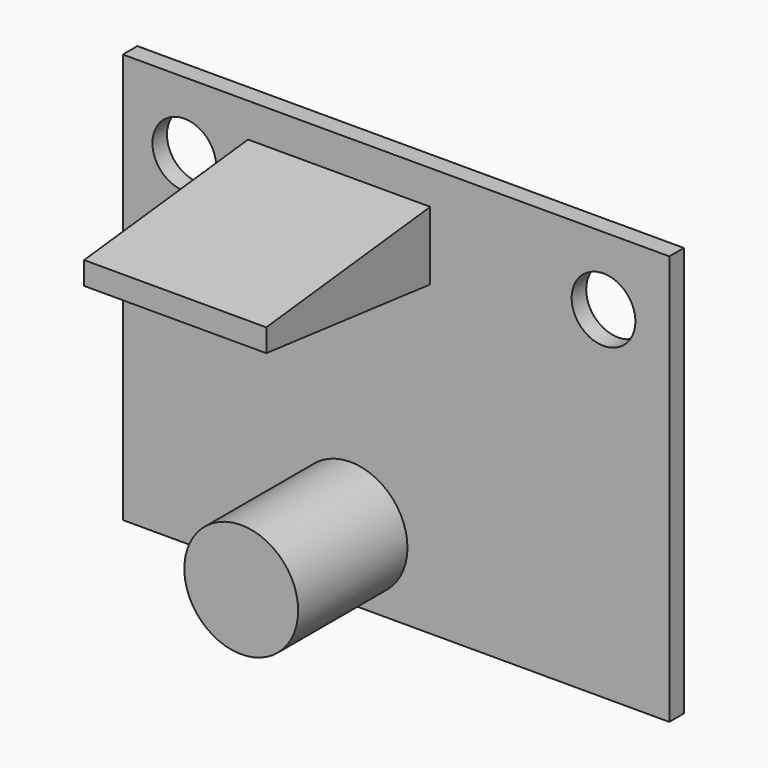
from build123d import *

# Parameters (mm, degrees)
F0_W     = 24
F0_H     = 18
F0_R     = 2.5
F0_W_2   = 8
F0_H_2   = 3
F1_DEPTH = 0.8
F2_D     = 2.8
F3_DEPTH = 2
F4_SIZE2 = 1.99999
F4_SIZE  = 0.99999
F5_SIZE2 = 0.99999
F5_SIZE  = 1.99999
F6_DEPTH = 6.8
F7_DEPTH = 9.8
F8_SIZE2 = 8.99999
F8_SIZE  = 0.99999


# Not quite as in the source:
# - a fillet or chamfer is up to 0.001 mm smaller than in the source, because OpenCascade refuses the exact size


with BuildPart() as f1:
    # F0 (on Front) → F1 (new body)
    with BuildSketch(Plane.XZ):
        Rectangle(F0_W, F0_H)
        with Locations((-2, -6)):
            Circle(F0_R, mode=Mode.SUBTRACT)
        with Locations((-2.5, 6)):
            Rectangle(F0_W_2, F0_H_2, mode=Mode.SUBTRACT)
        with Locations((-2.5, 6)):
            Rectangle(F0_W_2, F0_H_2)
        with Locations((-2, -6)):
            Circle(F0_R)
    extrude(amount=F1_DEPTH)

    # F2 (through all)
    with Locations(Plane(origin=(0, 0, 0), x_dir=(1, 0, 0), z_dir=(0, 1, 0))):
        with Locations((-9.3, -6), (9.11, -6)):
            Hole(F2_D / 2)

    # F0 (on Front) → F3 (join)
    with BuildSketch(Plane.XZ):
        with Locations((-2.5, 6)):
            Rectangle(F0_W_2, F0_H_2)
        with Locations((-2, -6)):
            Circle(F0_R)
    extrude(amount=-F3_DEPTH)

    # F4 (size 1 and 2 in the source; OpenCascade refuses exactly that, so slightly less here)
    f4_edges = [f1.edges().sort_by_distance(p)[0] for p in [
        (-2.5, 2, 4.5),
        (-2.5, 2, 7.5),
    ]]
    f4_side = f1.faces().sort_by_distance((-2.5, 2, 6))[0]
    chamfer(f4_edges, length=F4_SIZE, length2=F4_SIZE2, reference=f4_side)

    # F5 (size 2 and 1 in the source; OpenCascade refuses exactly that, so slightly less here)
    f5_edges = [f1.edges().sort_by_distance(p)[0] for p in [
        (-4.5, 2, -6),
    ]]
    f5_side = f1.faces().sort_by_distance((-4.5, 1, -6))[0]
    chamfer(f5_edges, length=F5_SIZE, length2=F5_SIZE2, reference=f5_side)

    # F0 (on Front) → F6 (join)
    with BuildSketch(Plane.XZ):
        with Locations((-2, -6)):
            Circle(F0_R)
    extrude(amount=F6_DEPTH)

    # F0 (on Front) → F7 (join)
    with BuildSketch(Plane.XZ):
        with Locations((-2.5, 6)):
            Rectangle(F0_W_2, F0_H_2)
    extrude(amount=F7_DEPTH)

    # F8 (size 1 and 9 in the source; OpenCascade refuses exactly that, so slightly less here)
    f8_edges = [f1.edges().sort_by_distance(p)[0] for p in [
        (-2.5, -9.8, 7.5),
        (-2.5, -9.8, 4.5),
    ]]
    f8_side = f1.faces().sort_by_distance((-2.5, -9.8, 6))[0]
    chamfer(f8_edges, length=F8_SIZE, length2=F8_SIZE2, reference=f8_side)


solid = f1.part
